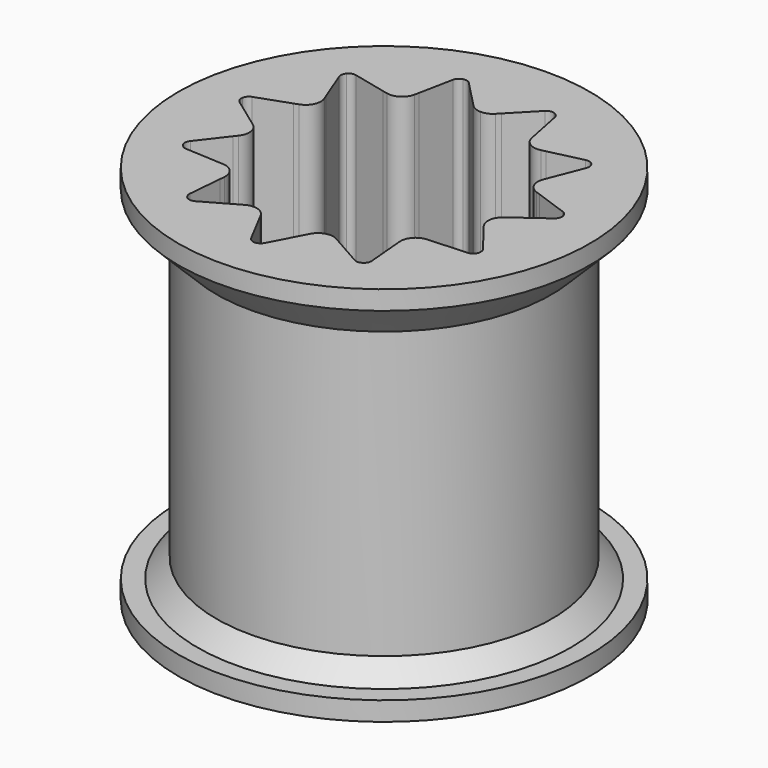
from build123d import *

# Parameters (mm, degrees)
F0_R     = 12.7
F0_R_2   = 4.318
F1_DEPTH = 11.43
F5_SIZE  = 1.5875
F7_DEPTH = 20.32
F8_DEPTH = 20.32


with BuildPart() as f1:
    # F0 (on Top) → F1 (new body)
    with BuildSketch(Plane.XY):
        Circle(F0_R)
        Circle(F0_R_2, mode=Mode.SUBTRACT)
    extrude(amount=F1_DEPTH)

    # F2 (on Front) → F3 (revolve)
    with BuildSketch(Plane.XZ):
        Polygon((-17.145, 0), (-7.62, 0), (-7.62, 1.5875), (-10.795, 1.5875), (-10.795, 31.75), (-17.145, 31.75), (-17.145, 30.1625), (-13.97, 30.1625), (-13.97, 26.9875), (-13.97, 1.5875), (-17.145, 1.5875), align=None)
        Polygon((-17.145, 30.1625), (-13.97, 26.9875), (-13.97, 30.1625), align=None)
    revolve(axis=Axis((0, 0, 11.5776285529), (0, 0, 1)))

    # F5
    f5_edges = [f1.edges().sort_by_distance(p)[0] for p in [
        (13.97, 0, 1.5875),
    ]]
    chamfer(f5_edges, length=F5_SIZE)

    # F6 (on face) → F7 (cut, through all)
    with BuildSketch(Plane.XY.offset(31.75)):
        with BuildLine():
            Line((-10.4525954137, -2.6972716061), (-12.1988524903, -4.9530041056))
            ThreePointArc((-12.1988524903, -4.9530041056), (-11.4913314283, -4.7408549365), (-11.0617303864, -5.3417178727))
            ThreePointArc((-11.0617303864, -5.3417178727), (-11.2602854276, -5.8029562036), (-11.7317801436, -5.9757498234))
            Line((-11.7317801436, -5.9757498234), (-8.8834561601, -6.1332072892))
            ThreePointArc((-8.8834561601, -6.1332072892), (-9.8194773853, -4.4844050753), (-10.4525954137, -2.6972716061))
        make_face()
        with BuildLine():
            ThreePointArc((-12.1988524903, -4.9530041056), (-12.3275224072, -5.2687355018), (-12.2743467257, -5.605506357))
            ThreePointArc((-12.2743467257, -5.605506357), (-12.0546549491, -5.8662319406), (-11.7317801436, -5.9757498234))
            ThreePointArc((-11.7317801436, -5.9757498234), (-11.2602854276, -5.8029562036), (-11.0617303864, -5.3417178727))
            ThreePointArc((-11.0617303864, -5.3417178727), (-11.4913314283, -4.7408549365), (-12.1988524903, -4.9530041056))
        make_face()
        with BuildLine():
            Line((-10.2515379451, 3.3820104613), (-12.9401239425, 2.4284653804))
            ThreePointArc((-12.9401239425, 2.4284653804), (-12.361504969, 2.3486470375), (-12.0928664774, 1.8299908459))
            ThreePointArc((-12.0928664774, 1.8299908459), (-12.4390464603, 1.264475154), (-13.1001357616, 1.3155585568))
            Line((-13.1001357616, 1.3155585568), (-10.7891010809, -0.3568232994))
            ThreePointArc((-10.7891010809, -0.3568232994), (-10.6851224667, 1.5362886683), (-10.2515379451, 3.3820104613))
        make_face()
        with BuildLine():
            ThreePointArc((-12.9401239425, 2.4284653804), (-13.2190652412, 2.2324194413), (-13.3564030838, 1.9203608324))
            ThreePointArc((-13.3564030838, 1.9203608324), (-13.3125454969, 1.5822501665), (-13.1001357616, 1.3155585568))
            ThreePointArc((-13.1001357616, 1.3155585568), (-12.4390464603, 1.264475154), (-12.0928664774, 1.8299908459))
            ThreePointArc((-12.0928664774, 1.8299908459), (-12.361504969, 2.3486470375), (-12.9401239425, 2.4284653804))
        make_face()
        with BuildLine():
            Line((-6.7956896128, 8.3875281035), (-9.5729974735, 9.0389142669))
            ThreePointArc((-9.5729974735, 9.0389142669), (-9.2203512646, 8.8151214081), (-9.0829948927, 8.4206904009))
            ThreePointArc((-9.0829948927, 8.4206904009), (-9.6001982975, 7.7967120663), (-10.3092908365, 8.1891863905))
            Line((-10.3092908365, 8.1891863905), (-9.2692826406, 5.5328495668))
            ThreePointArc((-9.2692826406, 5.5328495668), (-8.1583166623, 7.0692216147), (-6.7956896128, 8.3875281035))
        make_face()
        with BuildLine():
            ThreePointArc((-9.5729974735, 9.0389142669), (-9.9136482865, 9.0247969722), (-10.1978958619, 8.8365269791))
            ThreePointArc((-10.1978958619, 8.8365269791), (-10.3437969109, 8.5283789982), (-10.3092908365, 8.1891863905))
            ThreePointArc((-10.3092908365, 8.1891863905), (-9.6001982975, 7.7967120663), (-9.0829948927, 8.4206904009))
            ThreePointArc((-9.0829948927, 8.4206904009), (-9.2203512646, 8.8151214081), (-9.5729974735, 9.0389142669))
        make_face()
        with BuildLine():
            Line((-1.1822578445, 10.7300648362), (-3.1665119462, 12.7795717395))
            ThreePointArc((-3.1665119462, 12.7795717395), (-3.0341189729, 12.5761316197), (-2.9877285936, 12.3378802515))
            ThreePointArc((-2.9877285936, 12.3378802515), (-3.6854985998, 11.7059902877), (-4.2453189127, 12.4628054073))
            Line((-4.2453189127, 12.4628054073), (-4.8065324556, 9.6658817887))
            ThreePointArc((-4.8065324556, 9.6658817887), (-3.0413029616, 10.3577266471), (-1.1822578445, 10.7300648362))
        make_face()
        with BuildLine():
            ThreePointArc((-3.1665119462, 12.7795717395), (-3.4607180661, 12.9518652586), (-3.8016288198, 12.9471582743))
            ThreePointArc((-3.8016288198, 12.9471582743), (-4.090965925, 12.7668077529), (-4.2453189127, 12.4628054073))
            ThreePointArc((-4.2453189127, 12.4628054073), (-3.6854985998, 11.7059902877), (-2.9877285936, 12.3378802515))
            ThreePointArc((-2.9877285936, 12.3378802515), (-3.0341189729, 12.5761316197), (-3.1665119462, 12.7795717395))
        make_face()
        with BuildLine():
            Line((3.0413028854, 10.3577266695), (3.4438282673, 11.7286022581))
            ThreePointArc((3.4438282673, 11.7286022581), (3.008743441, 12.1758697278), (3.1665117699, 12.7795717652))
            Line((3.1665117699, 12.7795717652), (1.1822578227, 10.7300648386))
            ThreePointArc((1.1822578227, 10.7300648386), (2.1199705639, 10.5847886048), (3.0413028854, 10.3577266695))
        make_face()
        with BuildLine():
            ThreePointArc((4.2453187505, 12.462805481), (4.0909657389, 12.766807831), (3.8016286067, 12.9471583368))
            Line((3.8016286067, 12.9471583368), (3.4438282673, 11.7286022581))
            ThreePointArc((3.4438282673, 11.7286022581), (4.0032697568, 11.8295366107), (4.257728437, 12.3378802975))
            ThreePointArc((4.257728437, 12.3378802975), (4.2546183994, 12.4006503178), (4.2453187505, 12.462805481))
        make_face()
        with BuildLine():
            ThreePointArc((4.257728437, 12.3378802975), (4.0032697568, 11.8295366107), (3.4438282673, 11.7286022581))
            Line((3.4438282673, 11.7286022581), (3.0413028854, 10.3577266695))
            ThreePointArc((3.0413028854, 10.3577266695), (3.9391359635, 10.0506334557), (4.806532436, 9.6658817985))
            Line((4.806532436, 9.6658817985), (4.2453187505, 12.462805481))
            ThreePointArc((4.2453187505, 12.462805481), (4.2546183994, 12.4006503178), (4.257728437, 12.3378802975))
        make_face()
        with BuildLine():
            Line((3.4438282673, 11.7286022581), (3.8016286067, 12.9471583368))
            ThreePointArc((3.8016286067, 12.9471583368), (3.4607178673, 12.9518652935), (3.1665117699, 12.7795717652))
            ThreePointArc((3.1665117699, 12.7795717652), (3.008743441, 12.1758697278), (3.4438282673, 11.7286022581))
        make_face()
        with BuildLine():
            Line((-7.335027693, -7.9201889967), (-7.5845315655, -10.7619297844))
            ThreePointArc((-7.5845315655, -10.7619297844), (-6.924168837, -10.1830775705), (-6.3169650428, -10.8174689094))
            ThreePointArc((-6.3169650428, -10.8174689094), (-6.4032533172, -11.1370630929), (-6.6386672228, -11.3697998573))
            Line((-6.6386672228, -11.3697998573), (-4.157376676, -9.9623412998))
            ThreePointArc((-4.157376676, -9.9623412998), (-5.8362176152, -9.0813318928), (-7.335027693, -7.9201889967))
        make_face()
        with BuildLine():
            ThreePointArc((-7.5845315655, -10.7619297844), (-7.52207831, -11.0971041407), (-7.2952720168, -11.3516648675))
            ThreePointArc((-7.2952720168, -11.3516648675), (-6.969496637, -11.4522268501), (-6.6386672228, -11.3697998573))
            ThreePointArc((-6.6386672228, -11.3697998573), (-6.4032533172, -11.1370630929), (-6.3169650428, -10.8174689094))
            ThreePointArc((-6.3169650428, -10.8174689094), (-6.924168837, -10.1830775705), (-7.5845315655, -10.7619297844))
        make_face()
        with BuildLine():
            Line((-1.8886405066, -10.6285023421), (-0.5621754583, -13.1540187967))
            ThreePointArc((-0.5621754583, -13.1540187967), (-0.1520583482, -12.2422248716), (0.6350000816, -12.85875))
            ThreePointArc((0.6350000816, -12.85875), (0.6165252134, -13.0108084161), (0.5621756347, -13.1540187717))
            Line((0.5621756347, -13.1540187717), (1.8886405281, -10.6285023383))
            ThreePointArc((1.8886405281, -10.6285023383), (1.09e-08, -10.795), (-1.8886405066, -10.6285023421))
        make_face()
        with BuildLine():
            ThreePointArc((-0.5621754583, -13.1540187967), (-0.3284274706, -13.4022206459), (8.16e-08, -13.49375))
            ThreePointArc((8.16e-08, -13.49375), (0.3284276459, -13.4022206386), (0.5621756347, -13.1540187717))
            ThreePointArc((0.5621756347, -13.1540187717), (0.6165252134, -13.0108084161), (0.6350000816, -12.85875))
            ThreePointArc((0.6350000816, -12.85875), (-0.1520583482, -12.2422248716), (-0.5621754583, -13.1540187967))
        make_face()
        with BuildLine():
            Line((4.1573766962, -9.9623412914), (6.6386673847, -11.369799783))
            ThreePointArc((6.6386673847, -11.369799783), (6.6086582491, -10.2832728355), (7.5845317003, -10.7619296679))
            Line((7.5845317003, -10.7619296679), (7.3350277091, -7.9201889818))
            ThreePointArc((7.3350277091, -7.9201889818), (5.8362176336, -9.081331881), (4.1573766962, -9.9623412914))
        make_face()
        with BuildLine():
            ThreePointArc((6.6386673847, -11.369799783), (6.9694967855, -11.4522267615), (7.2952721492, -11.3516647824))
            ThreePointArc((7.2952721492, -11.3516647824), (7.5092913527, -11.1217919017), (7.5869651801, -10.8174688212))
            ThreePointArc((7.5869651801, -10.8174688212), (7.5863565184, -10.7896726012), (7.5845317003, -10.7619296679))
            ThreePointArc((7.5845317003, -10.7619296679), (6.6086582491, -10.2832728355), (6.6386673847, -11.369799783))
        make_face()
        with BuildLine():
            Line((8.8834561725, -6.1332072712), (11.7317802397, -5.9757496733))
            ThreePointArc((11.7317802397, -5.9757496733), (11.1191141312, -5.0779292038), (12.1988525408, -4.9530039347))
            Line((12.1988525408, -4.9530039347), (10.4525954192, -2.6972715849))
            ThreePointArc((10.4525954192, -2.6972715849), (9.8194773944, -4.4844050554), (8.8834561725, -6.1332072712))
        make_face()
        with BuildLine():
            ThreePointArc((11.7317802397, -5.9757496733), (12.0546550169, -5.866231792), (12.2743467819, -5.6055062342))
            ThreePointArc((12.2743467819, -5.6055062342), (12.3172187168, -5.4766966706), (12.3317304542, -5.3417177242))
            ThreePointArc((12.3317304542, -5.3417177242), (12.2975933857, -5.1363187527), (12.1988525408, -4.9530039347))
            ThreePointArc((12.1988525408, -4.9530039347), (11.1191141312, -5.0779292038), (11.7317802397, -5.9757496733))
        make_face()
        with BuildLine():
            ThreePointArc((13.1001357613, 1.315558735), (12.0993298406, 1.7396210711), (12.9401238926, 2.4284655514))
            Line((12.9401238926, 2.4284655514), (10.2515379382, 3.3820104821))
            ThreePointArc((10.2515379382, 3.3820104821), (10.6582685518, 1.7126985953), (10.795, 0))
            ThreePointArc((10.795, 0), (10.7935251696, -0.178436017), (10.7891010816, -0.3568232775))
            Line((10.7891010816, -0.3568232775), (13.1001357613, 1.315558735))
        make_face()
        with BuildLine():
            ThreePointArc((13.3628664542, 1.8299910074), (13.3612485452, 1.8752914129), (13.3564030629, 1.9203609777))
            ThreePointArc((13.3564030629, 1.9203609777), (13.2190652142, 2.2324196075), (12.9401238926, 2.4284655514))
            ThreePointArc((12.9401238926, 2.4284655514), (12.0993298406, 1.7396210711), (13.1001357613, 1.315558735))
            ThreePointArc((13.1001357613, 1.315558735), (13.2933821525, 1.541171003), (13.3628664542, 1.8299910074))
        make_face()
        with BuildLine():
            ThreePointArc((10.3092907399, 8.1891865402), (9.2380938153, 8.0048539475), (9.572997339, 9.0389143838))
            Line((9.572997339, 9.0389143838), (6.7956895958, 8.3875281173))
            ThreePointArc((6.7956895958, 8.3875281173), (8.158316648, 7.0692216312), (9.2692826294, 5.5328495856))
            Line((9.2692826294, 5.5328495856), (10.3092907399, 8.1891865402))
        make_face()
        with BuildLine():
            ThreePointArc((10.3529947858, 8.4206905243), (10.3129578717, 8.6426002501), (10.1978958049, 8.8365270449))
            ThreePointArc((10.1978958049, 8.8365270449), (9.9136482024, 9.0247970882), (9.572997339, 9.0389143838))
            ThreePointArc((9.572997339, 9.0389143838), (9.2380938153, 8.0048539475), (10.3092907399, 8.1891865402))
            ThreePointArc((10.3092907399, 8.1891865402), (10.3419731231, 8.302893943), (10.3529947858, 8.4206905243))
        make_face()
    extrude(amount=-F7_DEPTH, mode=Mode.SUBTRACT)

    # F4 (on face) → F8 (join, through all)
    with BuildSketch(Plane.XY.offset(11.43)):
        with BuildLine():
            Line((9.8859363825, 3.5116762306), (10.2515379382, 3.3820104821))
            ThreePointArc((10.2515379382, 3.3820104821), (9.8194773853, 4.4844050753), (9.2692826294, 5.5328495856))
            Line((9.2692826294, 5.5328495856), (9.1278593511, 5.1716332867))
            ThreePointArc((9.1278593511, 5.1716332867), (9.155218637, 4.1810482264), (9.8859363825, 3.5116762306))
        make_face()
        with BuildLine():
            ThreePointArc((10.4525954192, -2.6972715849), (10.6851224667, -1.5362886683), (10.7891010816, -0.3568232775))
            Line((10.7891010816, -0.3568232775), (10.474839974, -0.5842385682))
            ThreePointArc((10.474839974, -0.5842385682), (9.9623053531, -1.4323632965), (10.2151344151, -2.390530692))
            Line((10.2151344151, -2.390530692), (10.4525954192, -2.6972715849))
        make_face()
        with BuildLine():
            ThreePointArc((7.3350277091, -7.9201889818), (8.1583166623, -7.0692216147), (8.8834561725, -6.1332072712))
            Line((8.8834561725, -6.1332072712), (8.4961329169, -6.1546188058))
            ThreePointArc((8.4961329169, -6.1546188058), (7.6064305099, -6.5910095934), (7.3010994475, -7.5337610106))
            Line((7.3010994475, -7.5337610106), (7.3350277091, -7.9201889818))
        make_face()
        with BuildLine():
            ThreePointArc((1.8886405281, -10.6285023383), (3.0413029616, -10.3577266471), (4.1573766962, -9.9623412914))
            Line((4.1573766962, -9.9623412914), (3.8199636894, -9.770951059))
            ThreePointArc((3.8199636894, -9.770951059), (2.8355677243, -9.6570569142), (2.0690169925, -10.2850754393))
            Line((2.0690169925, -10.2850754393), (1.8886405281, -10.6285023383))
        make_face()
        with BuildLine():
            Line((-3.8199637387, -9.7709510869), (-4.157376676, -9.9623412998))
            ThreePointArc((-4.157376676, -9.9623412998), (-3.0413029406, -10.3577266533), (-1.8886405066, -10.6285023421))
            Line((-1.8886405066, -10.6285023421), (-2.0690170188, -10.2850753892))
            ThreePointArc((-2.0690170188, -10.2850753892), (-2.8355677786, -9.6570568982), (-3.8199637387, -9.7709510869))
        make_face()
        with BuildLine():
            Line((-8.4961329734, -6.1546188027), (-8.8834561601, -6.1332072892))
            ThreePointArc((-8.8834561601, -6.1332072892), (-8.158316648, -7.0692216312), (-7.335027693, -7.9201889967))
            Line((-7.335027693, -7.9201889967), (-7.3010994426, -7.5337609542))
            ThreePointArc((-7.3010994426, -7.5337609542), (-7.606430547, -6.5910095506), (-8.4961329734, -6.1546188027))
        make_face()
        with BuildLine():
            Line((-10.4748400199, -0.584238535), (-10.7891010809, -0.3568232994))
            ThreePointArc((-10.7891010809, -0.3568232994), (-10.6851224635, -1.53628869), (-10.4525954137, -2.6972716061))
            Line((-10.4525954137, -2.6972716061), (-10.2151343804, -2.3905306473))
            ThreePointArc((-10.2151343804, -2.3905306473), (-9.9623053612, -1.4323632405), (-10.4748400199, -0.584238535))
        make_face()
        with BuildLine():
            Line((-9.1278593717, 5.1716333395), (-9.2692826406, 5.5328495668))
            ThreePointArc((-9.2692826406, 5.5328495668), (-9.8194773944, 4.4844050554), (-10.2515379451, 3.3820104613))
            Line((-10.2515379451, 3.3820104613), (-9.8859363292, 3.5116762495))
            ThreePointArc((-9.8859363292, 3.5116762495), (-9.1552186135, 4.1810482779), (-9.1278593717, 5.1716333395))
        make_face()
        with BuildLine():
            Line((-4.8828478674, 9.2855481697), (-4.8065324556, 9.6658817887))
            ThreePointArc((-4.8065324556, 9.6658817887), (-5.8362176336, 9.081331881), (-6.7956896128, 8.3875281035))
            Line((-6.7956896128, 8.3875281035), (-6.4180233441, 8.2989507494))
            ThreePointArc((-6.4180233441, 8.2989507494), (-5.4414146437, 8.4670065099), (-4.8828478674, 9.2855481697))
        make_face()
        with BuildLine():
            Line((0, 10.06475), (0, 10.795))
            ThreePointArc((0, 10.795), (-0.592019887, 10.7787539843), (-1.1822578445, 10.7300648362))
            Line((-1.1822578445, 10.7300648362), (-0.9124332948, 10.4513670239))
            ThreePointArc((-0.9124332948, 10.4513670239), (-0.4954813924, 10.1653919753), (0, 10.06475))
        make_face()
        with BuildLine():
            ThreePointArc((1.1822578227, 10.7300648386), (0.5920198761, 10.7787539849), (0, 10.795))
            Line((0, 10.795), (0, 10.06475))
            ThreePointArc((0, 10.06475), (0.4954814184, 10.1653919864), (0.9124333342, 10.4513670646))
            Line((0.9124333342, 10.4513670646), (1.1822578227, 10.7300648386))
        make_face()
        with BuildLine():
            ThreePointArc((6.7956895958, 8.3875281173), (5.8362176152, 9.0813318928), (4.806532436, 9.6658817985))
            Line((4.806532436, 9.6658817985), (4.8828478786, 9.2855481142))
            ThreePointArc((4.8828478786, 9.2855481142), (5.4414146913, 8.4670064793), (6.4180233992, 8.2989507623))
            Line((6.4180233992, 8.2989507623), (6.7956895958, 8.3875281173))
        make_face()
    extrude(amount=F8_DEPTH)


solid = f1.part
